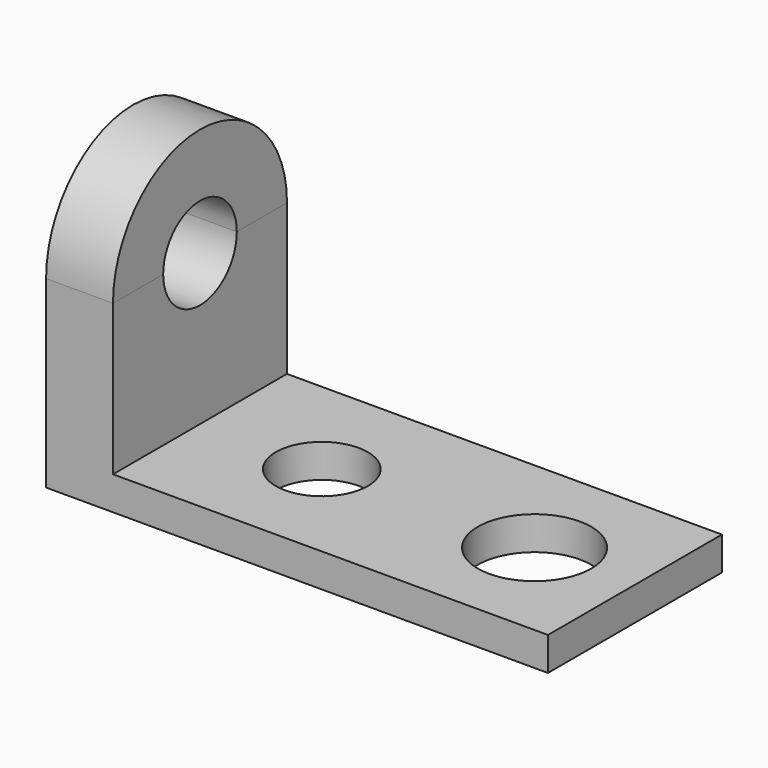
from build123d import *

# Parameters (mm, degrees)
F1_DEPTH = 82.55
F3_DEPTH = 25.4
F4_R     = 21.5178253772
F4_R_2   = 17.4625
F5_DEPTH = 25.4
F7_DEPTH = 25.4
F9_DEPTH = 25.4


with BuildPart() as f1:
    # F0 (on Front) → F1 (new body)
    with BuildSketch(Plane.XZ):
        Polygon((0, 69.85), (0, 0), (190.5, 0), (190.5, 12.7), (25.4, 12.7), (25.4, 69.85), align=None)
    extrude(amount=F1_DEPTH)

    # F4 (on face) → F5 (cut)
    with BuildSketch(Plane.XY.offset(12.7)):
        with Locations((152.4, -41.275)):
            Circle(F4_R)
        with Locations((71.6337114573, -41.275)):
            Circle(F4_R_2)
    extrude(amount=-F5_DEPTH, mode=Mode.SUBTRACT)

    # F6 (on face) → F7 (cut)
    with BuildSketch(Plane.YZ.offset(25.4)):
        with BuildLine():
            ThreePointArc((-58.7375, 69.85), (-41.275, 52.3875), (-23.8125, 69.85))
            Line((-23.8125, 69.85), (-58.7375, 69.85))
        make_face()
    extrude(amount=-F7_DEPTH, mode=Mode.SUBTRACT)


with BuildPart() as f3:
    # F2 (on face) → F3 (new body)
    with BuildSketch(Plane.YZ.offset(25.4)):
        with BuildLine():
            Line((-82.55, 69.85), (0, 69.85))
            ThreePointArc((0, 69.85), (-41.275, 111.125), (-82.55, 69.85))
        make_face()
    extrude(amount=-F3_DEPTH)

    # F8 (on face) → F9 (cut)
    with BuildSketch(Plane.YZ.offset(25.4)):
        with BuildLine():
            Line((-58.7375, 69.85), (-23.8125, 69.85))
            ThreePointArc((-23.8125, 69.85), (-41.275, 87.3125), (-58.7375, 69.85))
        make_face()
    extrude(amount=-F9_DEPTH, mode=Mode.SUBTRACT)


solid = Compound([f1.part, f3.part])
